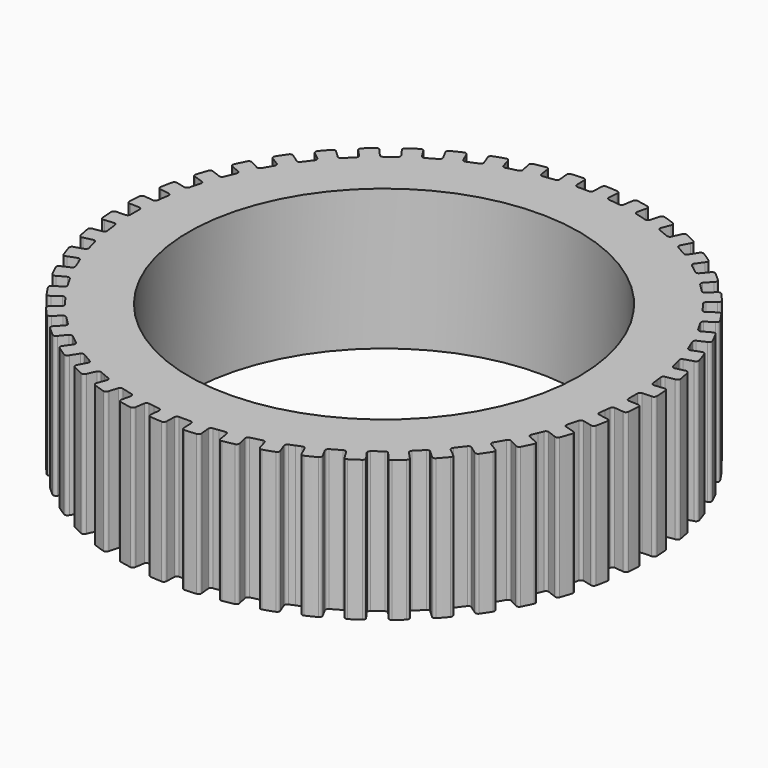
from build123d import *

# Parameters (mm, degrees)
F1_R     = 15
F1_R_2   = 11.1
F4_DEPTH = 8
F5_DEPTH = 8


# Not quite as in the source:
# - a feature names something its author has since deleted; it is built from what else it names


with BuildPart() as f4:
    # F1 (on Top) → F4 (new body)
    with BuildSketch(Plane.XY):
        Circle(F1_R)
        Circle(F1_R_2, mode=Mode.SUBTRACT)
    extrude(amount=F4_DEPTH)

    # F3 (on Top) + F2 (on Top) → F5 (cut)
    with BuildSketch(Plane.XY):
        with BuildLine():
            ThreePointArc((-14.6078107321, 2.4209827202), (-14.7318517717, 2.472566232), (-14.7728614863, 2.6004929356))
            Line((-14.7728614863, 2.6004929356), (-15.0180485763, 2.6327724283))
            Line((-15.0180485763, 2.6327724283), (-15.1877326262, 1.3438941086))
            Line((-15.1877326262, 1.3438941086), (-14.9425455361, 1.3116146158))
            ThreePointArc((-14.9425455361, 1.3116146158), (-14.8698233264, 1.4245682275), (-14.7366580875, 1.4422898902))
            Line((-14.7366580875, 1.4422898902), (-14.2148778682, 1.3912227941))
            ThreePointArc((-14.2148778682, 1.3912227941), (-14.1185132817, 1.4351704239), (-14.0707131699, 1.5296832643))
            Line((-14.0707131699, 1.5296832643), (-14.0289447884, 1.8469456199))
            Line((-14.0289447884, 1.8469456199), (-13.9871764069, 2.1642079756))
            ThreePointArc((-13.9871764069, 2.1642079756), (-14.0088860463, 2.2678719483), (-14.0905926055, 2.3352630891))
            Line((-14.0905926055, 2.3352630891), (-14.6078107321, 2.4209827202))
        make_face()
        with BuildLine():
            ThreePointArc((-13.4834652158, 6.1192693592), (-13.5899288642, 6.2011993888), (-13.5964313394, 6.3353811908))
            Line((-13.5964313394, 6.3353811908), (-13.8249093344, 6.4300198751))
            Line((-13.8249093344, 6.4300198751), (-14.3223977965, 5.2289764828))
            Line((-14.3223977965, 5.2289764828), (-14.0939198015, 5.1343377986))
            ThreePointArc((-14.0939198015, 5.1343377986), (-13.994440995, 5.2246207164), (-13.8612265478, 5.2072728282))
            Line((-13.8612265478, 5.2072728282), (-13.3704426953, 5.022899143))
            ThreePointArc((-13.3704426953, 5.022899143), (-13.265987169, 5.0404083034), (-13.1953540834, 5.1193291176))
            Line((-13.1953540834, 5.1193291176), (-13.072895385, 5.414970568))
            Line((-13.072895385, 5.414970568), (-12.9504366867, 5.7106120184))
            ThreePointArc((-12.9504366867, 5.7106120184), (-12.9445763776, 5.816362595), (-13.0060567426, 5.9026046521))
            Line((-13.0060567426, 5.9026046521), (-13.4834652158, 6.1192693592))
        make_face()
        with BuildLine():
            ThreePointArc((-14.4223273272, -3.3534707665), (-14.5566664602, -3.3532822666), (-14.6435099262, -3.2507871418))
            Line((-14.6435099262, -3.2507871418), (-14.8823860874, -3.3147938163))
            Line((-14.8823860874, -3.3147938163), (-14.5459213288, -4.5704973905))
            Line((-14.5459213288, -4.5704973905), (-14.3070451676, -4.506490716))
            ThreePointArc((-14.3070451676, -4.506490716), (-14.2830840823, -4.3743056012), (-14.1668372303, -4.306972789))
            Line((-14.1668372303, -4.306972789), (-13.6652326336, -4.1544759886))
            ThreePointArc((-13.6652326336, -4.1544759886), (-13.5930213943, -4.0769965423), (-13.5850283476, -3.9713857526))
            Line((-13.5850283476, -3.9713857526), (-13.667850442, -3.6622894882))
            Line((-13.667850442, -3.6622894882), (-13.7506725364, -3.3531932238))
            ThreePointArc((-13.7506725364, -3.3531932238), (-13.8104001128, -3.2657281204), (-13.9116766036, -3.2347345712))
            Line((-13.9116766036, -3.2347345712), (-14.4223273272, -3.3534707665))
        make_face()
        with BuildLine():
            ThreePointArc((-14.1668372303, 4.306972789), (-14.2830840823, 4.3743056012), (-14.3070451676, 4.506490716))
            Line((-14.3070451676, 4.506490716), (-14.5459213288, 4.5704973905))
            Line((-14.5459213288, 4.5704973905), (-14.8823860874, 3.3147938163))
            Line((-14.8823860874, 3.3147938163), (-14.6435099262, 3.2507871418))
            ThreePointArc((-14.6435099262, 3.2507871418), (-14.5566664602, 3.3532822666), (-14.4223273272, 3.3534707665))
            Line((-14.4223273272, 3.3534707665), (-13.9116766036, 3.2347345712))
            ThreePointArc((-13.9116766036, 3.2347345712), (-13.8104001128, 3.2657281204), (-13.7506725364, 3.3531932238))
            Line((-13.7506725364, 3.3531932238), (-13.667850442, 3.6622894882))
            Line((-13.667850442, 3.6622894882), (-13.5850283476, 3.9713857526))
            ThreePointArc((-13.5850283476, 3.9713857526), (-13.5930213943, 4.0769965423), (-13.6652326336, 4.1544759886))
            Line((-13.6652326336, 4.1544759886), (-14.1668372303, 4.306972789))
        make_face()
        with BuildLine():
            ThreePointArc((-14.7366580875, -1.4422898902), (-14.8698233264, -1.4245682275), (-14.9425455361, -1.3116146158))
            Line((-14.9425455361, -1.3116146158), (-15.1877326262, -1.3438941086))
            Line((-15.1877326262, -1.3438941086), (-15.0180485763, -2.6327724283))
            Line((-15.0180485763, -2.6327724283), (-14.7728614863, -2.6004929356))
            ThreePointArc((-14.7728614863, -2.6004929356), (-14.7318517717, -2.472566232), (-14.6078107321, -2.4209827202))
            Line((-14.6078107321, -2.4209827202), (-14.0905926055, -2.3352630891))
            ThreePointArc((-14.0905926055, -2.3352630891), (-14.0088860463, -2.2678719483), (-13.9871764069, -2.1642079756))
            Line((-13.9871764069, -2.1642079756), (-14.0289447884, -1.8469456199))
            Line((-14.0289447884, -1.8469456199), (-14.0707131699, -1.5296832643))
            ThreePointArc((-14.0707131699, -1.5296832643), (-14.1185132817, -1.4351704239), (-14.2148778682, -1.3912227941))
            Line((-14.2148778682, -1.3912227941), (-14.7366580875, -1.4422898902))
        make_face()
        with BuildLine():
            ThreePointArc((-14.7988405421, 0.4935689659), (-14.9285533928, 0.528520569), (-14.9859100491, 0.65))
            Line((-14.9859100491, 0.65), (-15.2332128489, 0.65))
            Line((-15.2332128489, 0.65), (-15.2332128489, -0.65))
            Line((-15.2332128489, -0.65), (-14.9859100491, -0.65))
            ThreePointArc((-14.9859100491, -0.65), (-14.9285533928, -0.528520569), (-14.7988405421, -0.4935689659))
            Line((-14.7988405421, -0.4935689659), (-14.2748586313, -0.4760931908))
            ThreePointArc((-14.2748586313, -0.4760931908), (-14.185054774, -0.4199434365), (-14.15, -0.32))
            Line((-14.15, -0.32), (-14.15, 0))
            Line((-14.15, 0), (-14.15, 0.32))
            ThreePointArc((-14.15, 0.32), (-14.185054774, 0.4199434365), (-14.2748586313, 0.4760931908))
            Line((-14.2748586313, 0.4760931908), (-14.7988405421, 0.4935689659))
        make_face()
        with BuildLine():
            ThreePointArc((-11.4402438275, 9.4005379039), (-11.5218747631, 9.5072310552), (-11.4934268659, 9.6385236877))
            Line((-11.4934268659, 9.6385236877), (-11.6896253682, 9.7890720935))
            Line((-11.6896253682, 9.7890720935), (-12.4810152259, 8.7577127511))
            Line((-12.4810152259, 8.7577127511), (-12.2848167236, 8.6071643453))
            ThreePointArc((-12.2848167236, 8.6071643453), (-12.1653606367, 8.6686239376), (-12.0411753256, 8.6173887283))
            Line((-12.0411753256, 8.6173887283), (-11.6148339485, 8.3122732161))
            ThreePointArc((-11.6148339485, 8.3122732161), (-11.5094059537, 8.3021506867), (-11.4207534224, 8.3601011516))
            Line((-11.4207534224, 8.3601011516), (-11.2259497651, 8.6139742205))
            Line((-11.2259497651, 8.6139742205), (-11.0311461078, 8.8678472894))
            ThreePointArc((-11.0311461078, 8.8678472894), (-10.9981152207, 8.9684777429), (-11.0351796062, 9.0676934625))
            Line((-11.0351796062, 9.0676934625), (-11.4402438275, 9.4005379039))
        make_face()
        with BuildLine():
            ThreePointArc((-10.1153545383, 10.8133664638), (-10.182360859, 10.9298018157), (-10.1370192102, 11.0562580257))
            Line((-10.1370192102, 11.0562580257), (-10.3118886969, 11.2311275125))
            Line((-10.3118886969, 11.2311275125), (-11.2311275125, 10.3118886969))
            Line((-11.2311275125, 10.3118886969), (-11.0562580257, 10.1370192102))
            ThreePointArc((-11.0562580257, 10.1370192102), (-10.9298018157, 10.182360859), (-10.8133664638, 10.1153545383))
            Line((-10.8133664638, 10.1153545383), (-10.4304980623, 9.757200615))
            ThreePointArc((-10.4304980623, 9.757200615), (-10.3272932739, 9.7334035705), (-10.2318351238, 9.7792867838))
            Line((-10.2318351238, 9.7792867838), (-10.0055609538, 10.0055609538))
            Line((-10.0055609538, 10.0055609538), (-9.7792867838, 10.2318351238))
            ThreePointArc((-9.7792867838, 10.2318351238), (-9.7334035705, 10.3272932739), (-9.757200615, 10.4304980623))
            Line((-9.757200615, 10.4304980623), (-10.1153545383, 10.8133664638))
        make_face()
        with BuildLine():
            ThreePointArc((-12.5693873731, 7.8268635341), (-12.6642461954, 7.9219889356), (-12.6531788014, 8.055871537))
            Line((-12.6531788014, 8.055871537), (-12.8673493084, 8.1795229369))
            Line((-12.8673493084, 8.1795229369), (-13.5173493084, 7.053689912))
            Line((-13.5173493084, 7.053689912), (-13.3031788014, 6.9300385121))
            ThreePointArc((-13.3031788014, 6.9300385121), (-13.1927667644, 7.0065644572), (-13.062956339, 6.9719770081))
            Line((-13.062956339, 6.9719770081), (-12.6004368055, 6.7251205179))
            ThreePointArc((-12.6004368055, 6.7251205179), (-12.4945895066, 6.7288457028), (-12.4142594635, 6.7978718708))
            Line((-12.4142594635, 6.7978718708), (-12.2542594635, 7.075))
            Line((-12.2542594635, 7.075), (-12.0942594635, 7.3521281292))
            ThreePointArc((-12.0942594635, 7.3521281292), (-12.0746460701, 7.4562090712), (-12.1243436147, 7.5497381134))
            Line((-12.1243436147, 7.5497381134), (-12.5693873731, 7.8268635341))
        make_face()
        with BuildLine():
            ThreePointArc((-8.6173887283, 12.0411753256), (-8.6686239376, 12.1653606367), (-8.6071643453, 12.2848167236))
            Line((-8.6071643453, 12.2848167236), (-8.7577127511, 12.4810152259))
            Line((-8.7577127511, 12.4810152259), (-9.7890720935, 11.6896253682))
            Line((-9.7890720935, 11.6896253682), (-9.6385236877, 11.4934268659))
            ThreePointArc((-9.6385236877, 11.4934268659), (-9.5072310552, 11.5218747631), (-9.4005379039, 11.4402438275))
            Line((-9.4005379039, 11.4402438275), (-9.0676934625, 11.0351796062))
            ThreePointArc((-9.0676934625, 11.0351796062), (-8.9684777429, 10.9981152207), (-8.8678472894, 11.0311461078))
            Line((-8.8678472894, 11.0311461078), (-8.6139742205, 11.2259497651))
            Line((-8.6139742205, 11.2259497651), (-8.3601011516, 11.4207534224))
            ThreePointArc((-8.3601011516, 11.4207534224), (-8.3021506867, 11.5094059537), (-8.3122732161, 11.6148339485))
            Line((-8.3122732161, 11.6148339485), (-8.6173887283, 12.0411753256))
        make_face()
        with BuildLine():
            ThreePointArc((-6.9719770081, 13.062956339), (-7.0065644572, 13.1927667644), (-6.9300385121, 13.3031788014))
            Line((-6.9300385121, 13.3031788014), (-7.053689912, 13.5173493084))
            Line((-7.053689912, 13.5173493084), (-8.1795229369, 12.8673493084))
            Line((-8.1795229369, 12.8673493084), (-8.055871537, 12.6531788014))
            ThreePointArc((-8.055871537, 12.6531788014), (-7.9219889356, 12.6642461954), (-7.8268635341, 12.5693873731))
            Line((-7.8268635341, 12.5693873731), (-7.5497381134, 12.1243436147))
            ThreePointArc((-7.5497381134, 12.1243436147), (-7.4562090712, 12.0746460701), (-7.3521281292, 12.0942594635))
            Line((-7.3521281292, 12.0942594635), (-7.075, 12.2542594635))
            Line((-7.075, 12.2542594635), (-6.7978718708, 12.4142594635))
            ThreePointArc((-6.7978718708, 12.4142594635), (-6.7288457028, 12.4945895066), (-6.7251205179, 12.6004368055))
            Line((-6.7251205179, 12.6004368055), (-6.9719770081, 13.062956339))
        make_face()
        with BuildLine():
            ThreePointArc((-5.2072728282, 13.8612265478), (-5.2246207164, 13.994440995), (-5.1343377986, 14.0939198015))
            Line((-5.1343377986, 14.0939198015), (-5.2289764828, 14.3223977965))
            Line((-5.2289764828, 14.3223977965), (-6.4300198751, 13.8249093344))
            Line((-6.4300198751, 13.8249093344), (-6.3353811908, 13.5964313394))
            ThreePointArc((-6.3353811908, 13.5964313394), (-6.2011993888, 13.5899288642), (-6.1192693592, 13.4834652158))
            Line((-6.1192693592, 13.4834652158), (-5.9026046521, 13.0060567426))
            ThreePointArc((-5.9026046521, 13.0060567426), (-5.816362595, 12.9445763776), (-5.7106120184, 12.9504366867))
            Line((-5.7106120184, 12.9504366867), (-5.414970568, 13.072895385))
            Line((-5.414970568, 13.072895385), (-5.1193291176, 13.1953540834))
            ThreePointArc((-5.1193291176, 13.1953540834), (-5.0404083034, 13.265987169), (-5.022899143, 13.3704426953))
            Line((-5.022899143, 13.3704426953), (-5.2072728282, 13.8612265478))
        make_face()
        with BuildLine():
            ThreePointArc((-1.4422898902, 14.7366580875), (-1.4245682275, 14.8698233264), (-1.3116146158, 14.9425455361))
            Line((-1.3116146158, 14.9425455361), (-1.3438941086, 15.1877326262))
            Line((-1.3438941086, 15.1877326262), (-2.6327724283, 15.0180485763))
            Line((-2.6327724283, 15.0180485763), (-2.6004929356, 14.7728614863))
            ThreePointArc((-2.6004929356, 14.7728614863), (-2.472566232, 14.7318517717), (-2.4209827202, 14.6078107321))
            Line((-2.4209827202, 14.6078107321), (-2.3352630891, 14.0905926055))
            ThreePointArc((-2.3352630891, 14.0905926055), (-2.2678719483, 14.0088860463), (-2.1642079756, 13.9871764069))
            Line((-2.1642079756, 13.9871764069), (-1.8469456199, 14.0289447884))
            Line((-1.8469456199, 14.0289447884), (-1.5296832643, 14.0707131699))
            ThreePointArc((-1.5296832643, 14.0707131699), (-1.4351704239, 14.1185132817), (-1.3912227941, 14.2148778682))
            Line((-1.3912227941, 14.2148778682), (-1.4422898902, 14.7366580875))
        make_face()
        with BuildLine():
            ThreePointArc((-3.3534707665, 14.4223273272), (-3.3532822666, 14.5566664602), (-3.2507871418, 14.6435099262))
            Line((-3.2507871418, 14.6435099262), (-3.3147938163, 14.8823860874))
            Line((-3.3147938163, 14.8823860874), (-4.5704973905, 14.5459213288))
            Line((-4.5704973905, 14.5459213288), (-4.506490716, 14.3070451676))
            ThreePointArc((-4.506490716, 14.3070451676), (-4.3743056012, 14.2830840823), (-4.306972789, 14.1668372303))
            Line((-4.306972789, 14.1668372303), (-4.1544759886, 13.6652326336))
            ThreePointArc((-4.1544759886, 13.6652326336), (-4.0769965423, 13.5930213943), (-3.9713857526, 13.5850283476))
            Line((-3.9713857526, 13.5850283476), (-3.6622894882, 13.667850442))
            Line((-3.6622894882, 13.667850442), (-3.3531932238, 13.7506725364))
            ThreePointArc((-3.3531932238, 13.7506725364), (-3.2657281204, 13.8104001128), (-3.2347345712, 13.9116766036))
            Line((-3.2347345712, 13.9116766036), (-3.3534707665, 14.4223273272))
        make_face()
        with BuildLine():
            Line((7.5497381134, 12.1243436147), (7.8268635341, 12.5693873731))
            ThreePointArc((7.8268635341, 12.5693873731), (7.9219889356, 12.6642461954), (8.055871537, 12.6531788014))
            Line((8.055871537, 12.6531788014), (8.1795229369, 12.8673493084))
            Line((8.1795229369, 12.8673493084), (7.053689912, 13.5173493084))
            Line((7.053689912, 13.5173493084), (6.9300385121, 13.3031788014))
            ThreePointArc((6.9300385121, 13.3031788014), (7.0065644572, 13.1927667644), (6.9719770081, 13.062956339))
            Line((6.9719770081, 13.062956339), (6.7251205179, 12.6004368055))
            ThreePointArc((6.7251205179, 12.6004368055), (6.7288457028, 12.4945895066), (6.7978718708, 12.4142594635))
            Line((6.7978718708, 12.4142594635), (7.075, 12.2542594635))
            Line((7.075, 12.2542594635), (7.3521281292, 12.0942594635))
            ThreePointArc((7.3521281292, 12.0942594635), (7.4562090712, 12.0746460701), (7.5497381134, 12.1243436147))
        make_face()
        with BuildLine():
            Line((10.4304980623, 9.757200615), (10.8133664638, 10.1153545383))
            ThreePointArc((10.8133664638, 10.1153545383), (10.9298018157, 10.182360859), (11.0562580257, 10.1370192102))
            Line((11.0562580257, 10.1370192102), (11.2311275125, 10.3118886969))
            Line((11.2311275125, 10.3118886969), (10.3118886969, 11.2311275125))
            Line((10.3118886969, 11.2311275125), (10.1370192102, 11.0562580257))
            ThreePointArc((10.1370192102, 11.0562580257), (10.182360859, 10.9298018157), (10.1153545383, 10.8133664638))
            Line((10.1153545383, 10.8133664638), (9.757200615, 10.4304980623))
            ThreePointArc((9.757200615, 10.4304980623), (9.7334035705, 10.3272932739), (9.7792867838, 10.2318351238))
            Line((9.7792867838, 10.2318351238), (10.0055609538, 10.0055609538))
            Line((10.0055609538, 10.0055609538), (10.2318351238, 9.7792867838))
            ThreePointArc((10.2318351238, 9.7792867838), (10.3272932739, 9.7334035705), (10.4304980623, 9.757200615))
        make_face()
        with BuildLine():
            Line((12.6004368055, 6.7251205179), (13.062956339, 6.9719770081))
            ThreePointArc((13.062956339, 6.9719770081), (13.1927667644, 7.0065644572), (13.3031788014, 6.9300385121))
            Line((13.3031788014, 6.9300385121), (13.5173493084, 7.053689912))
            Line((13.5173493084, 7.053689912), (12.8673493084, 8.1795229369))
            Line((12.8673493084, 8.1795229369), (12.6531788014, 8.055871537))
            ThreePointArc((12.6531788014, 8.055871537), (12.6642461954, 7.9219889356), (12.5693873731, 7.8268635341))
            Line((12.5693873731, 7.8268635341), (12.1243436147, 7.5497381134))
            ThreePointArc((12.1243436147, 7.5497381134), (12.0746460701, 7.4562090712), (12.0942594635, 7.3521281292))
            Line((12.0942594635, 7.3521281292), (12.2542594635, 7.075))
            Line((12.2542594635, 7.075), (12.4142594635, 6.7978718708))
            ThreePointArc((12.4142594635, 6.7978718708), (12.4945895066, 6.7288457028), (12.6004368055, 6.7251205179))
        make_face()
        with BuildLine():
            Line((9.0676934625, 11.0351796062), (9.4005379039, 11.4402438275))
            ThreePointArc((9.4005379039, 11.4402438275), (9.5072310552, 11.5218747631), (9.6385236877, 11.4934268659))
            Line((9.6385236877, 11.4934268659), (9.7890720935, 11.6896253682))
            Line((9.7890720935, 11.6896253682), (8.7577127511, 12.4810152259))
            Line((8.7577127511, 12.4810152259), (8.6071643453, 12.2848167236))
            ThreePointArc((8.6071643453, 12.2848167236), (8.6686239376, 12.1653606367), (8.6173887283, 12.0411753256))
            Line((8.6173887283, 12.0411753256), (8.3122732161, 11.6148339485))
            ThreePointArc((8.3122732161, 11.6148339485), (8.3021506867, 11.5094059537), (8.3601011516, 11.4207534224))
            Line((8.3601011516, 11.4207534224), (8.6139742205, 11.2259497651))
            Line((8.6139742205, 11.2259497651), (8.8678472894, 11.0311461078))
            ThreePointArc((8.8678472894, 11.0311461078), (8.9684777429, 10.9981152207), (9.0676934625, 11.0351796062))
        make_face()
        with BuildLine():
            Line((13.3704426953, 5.022899143), (13.8612265478, 5.2072728282))
            ThreePointArc((13.8612265478, 5.2072728282), (13.994440995, 5.2246207164), (14.0939198015, 5.1343377986))
            Line((14.0939198015, 5.1343377986), (14.3223977965, 5.2289764828))
            Line((14.3223977965, 5.2289764828), (13.8249093344, 6.4300198751))
            Line((13.8249093344, 6.4300198751), (13.5964313394, 6.3353811908))
            ThreePointArc((13.5964313394, 6.3353811908), (13.5899288642, 6.2011993888), (13.4834652158, 6.1192693592))
            Line((13.4834652158, 6.1192693592), (13.0060567426, 5.9026046521))
            ThreePointArc((13.0060567426, 5.9026046521), (12.9445763776, 5.816362595), (12.9504366867, 5.7106120184))
            Line((12.9504366867, 5.7106120184), (13.072895385, 5.414970568))
            Line((13.072895385, 5.414970568), (13.1953540834, 5.1193291176))
            ThreePointArc((13.1953540834, 5.1193291176), (13.265987169, 5.0404083034), (13.3704426953, 5.022899143))
        make_face()
        with BuildLine():
            Line((11.6148339485, 8.3122732161), (12.0411753256, 8.6173887283))
            ThreePointArc((12.0411753256, 8.6173887283), (12.1653606367, 8.6686239376), (12.2848167236, 8.6071643453))
            Line((12.2848167236, 8.6071643453), (12.4810152259, 8.7577127511))
            Line((12.4810152259, 8.7577127511), (11.6896253682, 9.7890720935))
            Line((11.6896253682, 9.7890720935), (11.4934268659, 9.6385236877))
            ThreePointArc((11.4934268659, 9.6385236877), (11.5218747631, 9.5072310552), (11.4402438275, 9.4005379039))
            Line((11.4402438275, 9.4005379039), (11.0351796062, 9.0676934625))
            ThreePointArc((11.0351796062, 9.0676934625), (10.9981152207, 8.9684777429), (11.0311461078, 8.8678472894))
            Line((11.0311461078, 8.8678472894), (11.2259497651, 8.6139742205))
            Line((11.2259497651, 8.6139742205), (11.4207534224, 8.3601011516))
            ThreePointArc((11.4207534224, 8.3601011516), (11.5094059537, 8.3021506867), (11.6148339485, 8.3122732161))
        make_face()
        with BuildLine():
            Line((13.9116766036, 3.2347345712), (14.4223273272, 3.3534707665))
            ThreePointArc((14.4223273272, 3.3534707665), (14.5566664602, 3.3532822666), (14.6435099262, 3.2507871418))
            Line((14.6435099262, 3.2507871418), (14.8823860874, 3.3147938163))
            Line((14.8823860874, 3.3147938163), (14.5459213288, 4.5704973905))
            Line((14.5459213288, 4.5704973905), (14.3070451676, 4.506490716))
            ThreePointArc((14.3070451676, 4.506490716), (14.2830840823, 4.3743056012), (14.1668372303, 4.306972789))
            Line((14.1668372303, 4.306972789), (13.6652326336, 4.1544759886))
            ThreePointArc((13.6652326336, 4.1544759886), (13.5930213943, 4.0769965423), (13.5850283476, 3.9713857526))
            Line((13.5850283476, 3.9713857526), (13.667850442, 3.6622894882))
            Line((13.667850442, 3.6622894882), (13.7506725364, 3.3531932238))
            ThreePointArc((13.7506725364, 3.3531932238), (13.8104001128, 3.2657281204), (13.9116766036, 3.2347345712))
        make_face()
        with BuildLine():
            ThreePointArc((14.6078107321, -2.4209827202), (14.7318517717, -2.472566232), (14.7728614863, -2.6004929356))
            Line((14.7728614863, -2.6004929356), (15.0180485763, -2.6327724283))
            Line((15.0180485763, -2.6327724283), (15.1877326262, -1.3438941086))
            Line((15.1877326262, -1.3438941086), (14.9425455361, -1.3116146158))
            ThreePointArc((14.9425455361, -1.3116146158), (14.8698233264, -1.4245682275), (14.7366580875, -1.4422898902))
            Line((14.7366580875, -1.4422898902), (14.2148778682, -1.3912227941))
            ThreePointArc((14.2148778682, -1.3912227941), (14.1185132817, -1.4351704239), (14.0707131699, -1.5296832643))
            Line((14.0707131699, -1.5296832643), (14.0289447884, -1.8469456199))
            Line((14.0289447884, -1.8469456199), (13.9871764069, -2.1642079756))
            ThreePointArc((13.9871764069, -2.1642079756), (14.0088860463, -2.2678719483), (14.0905926055, -2.3352630891))
            Line((14.0905926055, -2.3352630891), (14.6078107321, -2.4209827202))
        make_face()
        with BuildLine():
            Line((14.2748586313, -0.4760931908), (14.7988405421, -0.4935689659))
            ThreePointArc((14.7988405421, -0.4935689659), (14.9285533928, -0.528520569), (14.9859100491, -0.65))
            Line((14.9859100491, -0.65), (15.2332128489, -0.65))
            Line((15.2332128489, -0.65), (15.2332128489, 0.65))
            Line((15.2332128489, 0.65), (14.9859100491, 0.65))
            ThreePointArc((14.9859100491, 0.65), (14.9285533928, 0.528520569), (14.7988405421, 0.4935689659))
            Line((14.7988405421, 0.4935689659), (14.2748586313, 0.4760931908))
            ThreePointArc((14.2748586313, 0.4760931908), (14.185054774, 0.4199434365), (14.15, 0.32))
            Line((14.15, 0.32), (14.15, 0))
            Line((14.15, 0), (14.15, -0.32))
            ThreePointArc((14.15, -0.32), (14.185054774, -0.4199434365), (14.2748586313, -0.4760931908))
        make_face()
        with BuildLine():
            Line((14.2148778682, 1.3912227941), (14.7366580875, 1.4422898902))
            ThreePointArc((14.7366580875, 1.4422898902), (14.8698233264, 1.4245682275), (14.9425455361, 1.3116146158))
            Line((14.9425455361, 1.3116146158), (15.1877326262, 1.3438941086))
            Line((15.1877326262, 1.3438941086), (15.0180485763, 2.6327724283))
            Line((15.0180485763, 2.6327724283), (14.7728614863, 2.6004929356))
            ThreePointArc((14.7728614863, 2.6004929356), (14.7318517717, 2.472566232), (14.6078107321, 2.4209827202))
            Line((14.6078107321, 2.4209827202), (14.0905926055, 2.3352630891))
            ThreePointArc((14.0905926055, 2.3352630891), (14.0088860463, 2.2678719483), (13.9871764069, 2.1642079756))
            Line((13.9871764069, 2.1642079756), (14.0289447884, 1.8469456199))
            Line((14.0289447884, 1.8469456199), (14.0707131699, 1.5296832643))
            ThreePointArc((14.0707131699, 1.5296832643), (14.1185132817, 1.4351704239), (14.2148778682, 1.3912227941))
        make_face()
        with BuildLine():
            ThreePointArc((-13.8612265478, -5.2072728282), (-13.994440995, -5.2246207164), (-14.0939198015, -5.1343377986))
            Line((-14.0939198015, -5.1343377986), (-14.3223977965, -5.2289764828))
            Line((-14.3223977965, -5.2289764828), (-13.8249093344, -6.4300198751))
            Line((-13.8249093344, -6.4300198751), (-13.5964313394, -6.3353811908))
            ThreePointArc((-13.5964313394, -6.3353811908), (-13.5899288642, -6.2011993888), (-13.4834652158, -6.1192693592))
            Line((-13.4834652158, -6.1192693592), (-13.0060567426, -5.9026046521))
            ThreePointArc((-13.0060567426, -5.9026046521), (-12.9445763776, -5.816362595), (-12.9504366867, -5.7106120184))
            Line((-12.9504366867, -5.7106120184), (-13.072895385, -5.414970568))
            Line((-13.072895385, -5.414970568), (-13.1953540834, -5.1193291176))
            ThreePointArc((-13.1953540834, -5.1193291176), (-13.265987169, -5.0404083034), (-13.3704426953, -5.022899143))
            Line((-13.3704426953, -5.022899143), (-13.8612265478, -5.2072728282))
        make_face()
        with BuildLine():
            ThreePointArc((-13.062956339, -6.9719770081), (-13.1927667644, -7.0065644572), (-13.3031788014, -6.9300385121))
            Line((-13.3031788014, -6.9300385121), (-13.5173493084, -7.053689912))
            Line((-13.5173493084, -7.053689912), (-12.8673493084, -8.1795229369))
            Line((-12.8673493084, -8.1795229369), (-12.6531788014, -8.055871537))
            ThreePointArc((-12.6531788014, -8.055871537), (-12.6642461954, -7.9219889356), (-12.5693873731, -7.8268635341))
            Line((-12.5693873731, -7.8268635341), (-12.1243436147, -7.5497381134))
            ThreePointArc((-12.1243436147, -7.5497381134), (-12.0746460701, -7.4562090712), (-12.0942594635, -7.3521281292))
            Line((-12.0942594635, -7.3521281292), (-12.2542594635, -7.075))
            Line((-12.2542594635, -7.075), (-12.4142594635, -6.7978718708))
            ThreePointArc((-12.4142594635, -6.7978718708), (-12.4945895066, -6.7288457028), (-12.6004368055, -6.7251205179))
            Line((-12.6004368055, -6.7251205179), (-13.062956339, -6.9719770081))
        make_face()
        with BuildLine():
            ThreePointArc((-12.0411753256, -8.6173887283), (-12.1653606367, -8.6686239376), (-12.2848167236, -8.6071643453))
            Line((-12.2848167236, -8.6071643453), (-12.4810152259, -8.7577127511))
            Line((-12.4810152259, -8.7577127511), (-11.6896253682, -9.7890720935))
            Line((-11.6896253682, -9.7890720935), (-11.4934268659, -9.6385236877))
            ThreePointArc((-11.4934268659, -9.6385236877), (-11.5218747631, -9.5072310552), (-11.4402438275, -9.4005379039))
            Line((-11.4402438275, -9.4005379039), (-11.0351796062, -9.0676934625))
            ThreePointArc((-11.0351796062, -9.0676934625), (-10.9981152207, -8.9684777429), (-11.0311461078, -8.8678472894))
            Line((-11.0311461078, -8.8678472894), (-11.2259497651, -8.6139742205))
            Line((-11.2259497651, -8.6139742205), (-11.4207534224, -8.3601011516))
            ThreePointArc((-11.4207534224, -8.3601011516), (-11.5094059537, -8.3021506867), (-11.6148339485, -8.3122732161))
            Line((-11.6148339485, -8.3122732161), (-12.0411753256, -8.6173887283))
        make_face()
        with BuildLine():
            ThreePointArc((-9.4005379039, -11.4402438275), (-9.5072310552, -11.5218747631), (-9.6385236877, -11.4934268659))
            Line((-9.6385236877, -11.4934268659), (-9.7890720935, -11.6896253682))
            Line((-9.7890720935, -11.6896253682), (-8.7577127511, -12.4810152259))
            Line((-8.7577127511, -12.4810152259), (-8.6071643453, -12.2848167236))
            ThreePointArc((-8.6071643453, -12.2848167236), (-8.6686239376, -12.1653606367), (-8.6173887283, -12.0411753256))
            Line((-8.6173887283, -12.0411753256), (-8.3122732161, -11.6148339485))
            ThreePointArc((-8.3122732161, -11.6148339485), (-8.3021506867, -11.5094059537), (-8.3601011516, -11.4207534224))
            Line((-8.3601011516, -11.4207534224), (-8.6139742205, -11.2259497651))
            Line((-8.6139742205, -11.2259497651), (-8.8678472894, -11.0311461078))
            ThreePointArc((-8.8678472894, -11.0311461078), (-8.9684777429, -10.9981152207), (-9.0676934625, -11.0351796062))
            Line((-9.0676934625, -11.0351796062), (-9.4005379039, -11.4402438275))
        make_face()
        with BuildLine():
            ThreePointArc((-7.8268635341, -12.5693873731), (-7.9219889356, -12.6642461954), (-8.055871537, -12.6531788014))
            Line((-8.055871537, -12.6531788014), (-8.1795229369, -12.8673493084))
            Line((-8.1795229369, -12.8673493084), (-7.053689912, -13.5173493084))
            Line((-7.053689912, -13.5173493084), (-6.9300385121, -13.3031788014))
            ThreePointArc((-6.9300385121, -13.3031788014), (-7.0065644572, -13.1927667644), (-6.9719770081, -13.062956339))
            Line((-6.9719770081, -13.062956339), (-6.7251205179, -12.6004368055))
            ThreePointArc((-6.7251205179, -12.6004368055), (-6.7288457028, -12.4945895066), (-6.7978718708, -12.4142594635))
            Line((-6.7978718708, -12.4142594635), (-7.075, -12.2542594635))
            Line((-7.075, -12.2542594635), (-7.3521281292, -12.0942594635))
            ThreePointArc((-7.3521281292, -12.0942594635), (-7.4562090712, -12.0746460701), (-7.5497381134, -12.1243436147))
            Line((-7.5497381134, -12.1243436147), (-7.8268635341, -12.5693873731))
        make_face()
        with BuildLine():
            ThreePointArc((-10.8133664638, -10.1153545383), (-10.9298018157, -10.182360859), (-11.0562580257, -10.1370192102))
            Line((-11.0562580257, -10.1370192102), (-11.2311275125, -10.3118886969))
            Line((-11.2311275125, -10.3118886969), (-10.3118886969, -11.2311275125))
            Line((-10.3118886969, -11.2311275125), (-10.1370192102, -11.0562580257))
            ThreePointArc((-10.1370192102, -11.0562580257), (-10.182360859, -10.9298018157), (-10.1153545383, -10.8133664638))
            Line((-10.1153545383, -10.8133664638), (-9.757200615, -10.4304980623))
            ThreePointArc((-9.757200615, -10.4304980623), (-9.7334035705, -10.3272932739), (-9.7792867838, -10.2318351238))
            Line((-9.7792867838, -10.2318351238), (-10.0055609538, -10.0055609538))
            Line((-10.0055609538, -10.0055609538), (-10.2318351238, -9.7792867838))
            ThreePointArc((-10.2318351238, -9.7792867838), (-10.3272932739, -9.7334035705), (-10.4304980623, -9.757200615))
            Line((-10.4304980623, -9.757200615), (-10.8133664638, -10.1153545383))
        make_face()
        with BuildLine():
            ThreePointArc((-6.1192693592, -13.4834652158), (-6.2011993888, -13.5899288642), (-6.3353811908, -13.5964313394))
            Line((-6.3353811908, -13.5964313394), (-6.4300198751, -13.8249093344))
            Line((-6.4300198751, -13.8249093344), (-5.2289764828, -14.3223977965))
            Line((-5.2289764828, -14.3223977965), (-5.1343377986, -14.0939198015))
            ThreePointArc((-5.1343377986, -14.0939198015), (-5.2246207164, -13.994440995), (-5.2072728282, -13.8612265478))
            Line((-5.2072728282, -13.8612265478), (-5.022899143, -13.3704426953))
            ThreePointArc((-5.022899143, -13.3704426953), (-5.0404083034, -13.265987169), (-5.1193291176, -13.1953540834))
            Line((-5.1193291176, -13.1953540834), (-5.414970568, -13.072895385))
            Line((-5.414970568, -13.072895385), (-5.7106120184, -12.9504366867))
            ThreePointArc((-5.7106120184, -12.9504366867), (-5.816362595, -12.9445763776), (-5.9026046521, -13.0060567426))
            Line((-5.9026046521, -13.0060567426), (-6.1192693592, -13.4834652158))
        make_face()
        with BuildLine():
            ThreePointArc((-4.306972789, -14.1668372303), (-4.3743056012, -14.2830840823), (-4.506490716, -14.3070451676))
            Line((-4.506490716, -14.3070451676), (-4.5704973905, -14.5459213288))
            Line((-4.5704973905, -14.5459213288), (-3.3147938163, -14.8823860874))
            Line((-3.3147938163, -14.8823860874), (-3.2507871418, -14.6435099262))
            ThreePointArc((-3.2507871418, -14.6435099262), (-3.3532822666, -14.5566664602), (-3.3534707665, -14.4223273272))
            Line((-3.3534707665, -14.4223273272), (-3.2347345712, -13.9116766036))
            ThreePointArc((-3.2347345712, -13.9116766036), (-3.2657281204, -13.8104001128), (-3.3531932238, -13.7506725364))
            Line((-3.3531932238, -13.7506725364), (-3.6622894882, -13.667850442))
            Line((-3.6622894882, -13.667850442), (-3.9713857526, -13.5850283476))
            ThreePointArc((-3.9713857526, -13.5850283476), (-4.0769965423, -13.5930213943), (-4.1544759886, -13.6652326336))
            Line((-4.1544759886, -13.6652326336), (-4.306972789, -14.1668372303))
        make_face()
        with BuildLine():
            ThreePointArc((-2.4209827202, -14.6078107321), (-2.472566232, -14.7318517717), (-2.6004929356, -14.7728614863))
            Line((-2.6004929356, -14.7728614863), (-2.6327724283, -15.0180485763))
            Line((-2.6327724283, -15.0180485763), (-1.3438941086, -15.1877326262))
            Line((-1.3438941086, -15.1877326262), (-1.3116146158, -14.9425455361))
            ThreePointArc((-1.3116146158, -14.9425455361), (-1.4245682275, -14.8698233264), (-1.4422898902, -14.7366580875))
            Line((-1.4422898902, -14.7366580875), (-1.3912227941, -14.2148778682))
            ThreePointArc((-1.3912227941, -14.2148778682), (-1.4351704239, -14.1185132817), (-1.5296832643, -14.0707131699))
            Line((-1.5296832643, -14.0707131699), (-1.8469456199, -14.0289447884))
            Line((-1.8469456199, -14.0289447884), (-2.1642079756, -13.9871764069))
            ThreePointArc((-2.1642079756, -13.9871764069), (-2.2678719483, -14.0088860463), (-2.3352630891, -14.0905926055))
            Line((-2.3352630891, -14.0905926055), (-2.4209827202, -14.6078107321))
        make_face()
        with BuildLine():
            ThreePointArc((-0.4935689659, -14.7988405421), (-0.528520569, -14.9285533928), (-0.65, -14.9859100491))
            Line((-0.65, -14.9859100491), (-0.65, -15.2332128489))
            Line((-0.65, -15.2332128489), (0.65, -15.2332128489))
            Line((0.65, -15.2332128489), (0.65, -14.9859100491))
            ThreePointArc((0.65, -14.9859100491), (0.528520569, -14.9285533928), (0.4935689659, -14.7988405421))
            Line((0.4935689659, -14.7988405421), (0.4760931908, -14.2748586313))
            ThreePointArc((0.4760931908, -14.2748586313), (0.4199434365, -14.185054774), (0.32, -14.15))
            Line((0.32, -14.15), (0, -14.15))
            Line((0, -14.15), (-0.32, -14.15))
            ThreePointArc((-0.32, -14.15), (-0.4199434365, -14.185054774), (-0.4760931908, -14.2748586313))
            Line((-0.4760931908, -14.2748586313), (-0.4935689659, -14.7988405421))
        make_face()
        with BuildLine():
            ThreePointArc((1.4422898902, -14.7366580875), (1.4245682275, -14.8698233264), (1.3116146158, -14.9425455361))
            Line((1.3116146158, -14.9425455361), (1.3438941086, -15.1877326262))
            Line((1.3438941086, -15.1877326262), (2.6327724283, -15.0180485763))
            Line((2.6327724283, -15.0180485763), (2.6004929356, -14.7728614863))
            ThreePointArc((2.6004929356, -14.7728614863), (2.472566232, -14.7318517717), (2.4209827202, -14.6078107321))
            Line((2.4209827202, -14.6078107321), (2.3352630891, -14.0905926055))
            ThreePointArc((2.3352630891, -14.0905926055), (2.2678719483, -14.0088860463), (2.1642079756, -13.9871764069))
            Line((2.1642079756, -13.9871764069), (1.8469456199, -14.0289447884))
            Line((1.8469456199, -14.0289447884), (1.5296832643, -14.0707131699))
            ThreePointArc((1.5296832643, -14.0707131699), (1.4351704239, -14.1185132817), (1.3912227941, -14.2148778682))
            Line((1.3912227941, -14.2148778682), (1.4422898902, -14.7366580875))
        make_face()
        with BuildLine():
            ThreePointArc((3.3534707665, -14.4223273272), (3.3532822666, -14.5566664602), (3.2507871418, -14.6435099262))
            Line((3.2507871418, -14.6435099262), (3.3147938163, -14.8823860874))
            Line((3.3147938163, -14.8823860874), (4.5704973905, -14.5459213288))
            Line((4.5704973905, -14.5459213288), (4.506490716, -14.3070451676))
            ThreePointArc((4.506490716, -14.3070451676), (4.3743056012, -14.2830840823), (4.306972789, -14.1668372303))
            Line((4.306972789, -14.1668372303), (4.1544759886, -13.6652326336))
            ThreePointArc((4.1544759886, -13.6652326336), (4.0769965423, -13.5930213943), (3.9713857526, -13.5850283476))
            Line((3.9713857526, -13.5850283476), (3.6622894882, -13.667850442))
            Line((3.6622894882, -13.667850442), (3.3531932238, -13.7506725364))
            ThreePointArc((3.3531932238, -13.7506725364), (3.2657281204, -13.8104001128), (3.2347345712, -13.9116766036))
            Line((3.2347345712, -13.9116766036), (3.3534707665, -14.4223273272))
        make_face()
        with BuildLine():
            ThreePointArc((5.2072728282, -13.8612265478), (5.2246207164, -13.994440995), (5.1343377986, -14.0939198015))
            Line((5.1343377986, -14.0939198015), (5.2289764828, -14.3223977965))
            Line((5.2289764828, -14.3223977965), (6.4300198751, -13.8249093344))
            Line((6.4300198751, -13.8249093344), (6.3353811908, -13.5964313394))
            ThreePointArc((6.3353811908, -13.5964313394), (6.2011993888, -13.5899288642), (6.1192693592, -13.4834652158))
            Line((6.1192693592, -13.4834652158), (5.9026046521, -13.0060567426))
            ThreePointArc((5.9026046521, -13.0060567426), (5.816362595, -12.9445763776), (5.7106120184, -12.9504366867))
            Line((5.7106120184, -12.9504366867), (5.414970568, -13.072895385))
            Line((5.414970568, -13.072895385), (5.1193291176, -13.1953540834))
            ThreePointArc((5.1193291176, -13.1953540834), (5.0404083034, -13.265987169), (5.022899143, -13.3704426953))
            Line((5.022899143, -13.3704426953), (5.2072728282, -13.8612265478))
        make_face()
        with BuildLine():
            ThreePointArc((6.9719770081, -13.062956339), (7.0065644572, -13.1927667644), (6.9300385121, -13.3031788014))
            Line((6.9300385121, -13.3031788014), (7.053689912, -13.5173493084))
            Line((7.053689912, -13.5173493084), (8.1795229369, -12.8673493084))
            Line((8.1795229369, -12.8673493084), (8.055871537, -12.6531788014))
            ThreePointArc((8.055871537, -12.6531788014), (7.9219889356, -12.6642461954), (7.8268635341, -12.5693873731))
            Line((7.8268635341, -12.5693873731), (7.5497381134, -12.1243436147))
            ThreePointArc((7.5497381134, -12.1243436147), (7.4562090712, -12.0746460701), (7.3521281292, -12.0942594635))
            Line((7.3521281292, -12.0942594635), (7.075, -12.2542594635))
            Line((7.075, -12.2542594635), (6.7978718708, -12.4142594635))
            ThreePointArc((6.7978718708, -12.4142594635), (6.7288457028, -12.4945895066), (6.7251205179, -12.6004368055))
            Line((6.7251205179, -12.6004368055), (6.9719770081, -13.062956339))
        make_face()
        with BuildLine():
            ThreePointArc((8.6173887283, -12.0411753256), (8.6686239376, -12.1653606367), (8.6071643453, -12.2848167236))
            Line((8.6071643453, -12.2848167236), (8.7577127511, -12.4810152259))
            Line((8.7577127511, -12.4810152259), (9.7890720935, -11.6896253682))
            Line((9.7890720935, -11.6896253682), (9.6385236877, -11.4934268659))
            ThreePointArc((9.6385236877, -11.4934268659), (9.5072310552, -11.5218747631), (9.4005379039, -11.4402438275))
            Line((9.4005379039, -11.4402438275), (9.0676934625, -11.0351796062))
            ThreePointArc((9.0676934625, -11.0351796062), (8.9684777429, -10.9981152207), (8.8678472894, -11.0311461078))
            Line((8.8678472894, -11.0311461078), (8.6139742205, -11.2259497651))
            Line((8.6139742205, -11.2259497651), (8.3601011516, -11.4207534224))
            ThreePointArc((8.3601011516, -11.4207534224), (8.3021506867, -11.5094059537), (8.3122732161, -11.6148339485))
            Line((8.3122732161, -11.6148339485), (8.6173887283, -12.0411753256))
        make_face()
        with BuildLine():
            ThreePointArc((10.1153545383, -10.8133664638), (10.182360859, -10.9298018157), (10.1370192102, -11.0562580257))
            Line((10.1370192102, -11.0562580257), (10.3118886969, -11.2311275125))
            Line((10.3118886969, -11.2311275125), (11.2311275125, -10.3118886969))
            Line((11.2311275125, -10.3118886969), (11.0562580257, -10.1370192102))
            ThreePointArc((11.0562580257, -10.1370192102), (10.9298018157, -10.182360859), (10.8133664638, -10.1153545383))
            Line((10.8133664638, -10.1153545383), (10.4304980623, -9.757200615))
            ThreePointArc((10.4304980623, -9.757200615), (10.3272932739, -9.7334035705), (10.2318351238, -9.7792867838))
            Line((10.2318351238, -9.7792867838), (10.0055609538, -10.0055609538))
            Line((10.0055609538, -10.0055609538), (9.7792867838, -10.2318351238))
            ThreePointArc((9.7792867838, -10.2318351238), (9.7334035705, -10.3272932739), (9.757200615, -10.4304980623))
            Line((9.757200615, -10.4304980623), (10.1153545383, -10.8133664638))
        make_face()
        with BuildLine():
            ThreePointArc((11.4402438275, -9.4005379039), (11.5218747631, -9.5072310552), (11.4934268659, -9.6385236877))
            Line((11.4934268659, -9.6385236877), (11.6896253682, -9.7890720935))
            Line((11.6896253682, -9.7890720935), (12.4810152259, -8.7577127511))
            Line((12.4810152259, -8.7577127511), (12.2848167236, -8.6071643453))
            ThreePointArc((12.2848167236, -8.6071643453), (12.1653606367, -8.6686239376), (12.0411753256, -8.6173887283))
            Line((12.0411753256, -8.6173887283), (11.6148339485, -8.3122732161))
            ThreePointArc((11.6148339485, -8.3122732161), (11.5094059537, -8.3021506867), (11.4207534224, -8.3601011516))
            Line((11.4207534224, -8.3601011516), (11.2259497651, -8.6139742205))
            Line((11.2259497651, -8.6139742205), (11.0311461078, -8.8678472894))
            ThreePointArc((11.0311461078, -8.8678472894), (10.9981152207, -8.9684777429), (11.0351796062, -9.0676934625))
            Line((11.0351796062, -9.0676934625), (11.4402438275, -9.4005379039))
        make_face()
        with BuildLine():
            ThreePointArc((12.5693873731, -7.8268635341), (12.6642461954, -7.9219889356), (12.6531788014, -8.055871537))
            Line((12.6531788014, -8.055871537), (12.8673493084, -8.1795229369))
            Line((12.8673493084, -8.1795229369), (13.5173493084, -7.053689912))
            Line((13.5173493084, -7.053689912), (13.3031788014, -6.9300385121))
            ThreePointArc((13.3031788014, -6.9300385121), (13.1927667644, -7.0065644572), (13.062956339, -6.9719770081))
            Line((13.062956339, -6.9719770081), (12.6004368055, -6.7251205179))
            ThreePointArc((12.6004368055, -6.7251205179), (12.4945895066, -6.7288457028), (12.4142594635, -6.7978718708))
            Line((12.4142594635, -6.7978718708), (12.2542594635, -7.075))
            Line((12.2542594635, -7.075), (12.0942594635, -7.3521281292))
            ThreePointArc((12.0942594635, -7.3521281292), (12.0746460701, -7.4562090712), (12.1243436147, -7.5497381134))
            Line((12.1243436147, -7.5497381134), (12.5693873731, -7.8268635341))
        make_face()
        with BuildLine():
            ThreePointArc((13.4834652158, -6.1192693592), (13.5899288642, -6.2011993888), (13.5964313394, -6.3353811908))
            Line((13.5964313394, -6.3353811908), (13.8249093344, -6.4300198751))
            Line((13.8249093344, -6.4300198751), (14.3223977965, -5.2289764828))
            Line((14.3223977965, -5.2289764828), (14.0939198015, -5.1343377986))
            ThreePointArc((14.0939198015, -5.1343377986), (13.994440995, -5.2246207164), (13.8612265478, -5.2072728282))
            Line((13.8612265478, -5.2072728282), (13.3704426953, -5.022899143))
            ThreePointArc((13.3704426953, -5.022899143), (13.265987169, -5.0404083034), (13.1953540834, -5.1193291176))
            Line((13.1953540834, -5.1193291176), (13.072895385, -5.414970568))
            Line((13.072895385, -5.414970568), (12.9504366867, -5.7106120184))
            ThreePointArc((12.9504366867, -5.7106120184), (12.9445763776, -5.816362595), (13.0060567426, -5.9026046521))
            Line((13.0060567426, -5.9026046521), (13.4834652158, -6.1192693592))
        make_face()
        with BuildLine():
            ThreePointArc((14.1668372303, -4.306972789), (14.2830840823, -4.3743056012), (14.3070451676, -4.506490716))
            Line((14.3070451676, -4.506490716), (14.5459213288, -4.5704973905))
            Line((14.5459213288, -4.5704973905), (14.8823860874, -3.3147938163))
            Line((14.8823860874, -3.3147938163), (14.6435099262, -3.2507871418))
            ThreePointArc((14.6435099262, -3.2507871418), (14.5566664602, -3.3532822666), (14.4223273272, -3.3534707665))
            Line((14.4223273272, -3.3534707665), (13.9116766036, -3.2347345712))
            ThreePointArc((13.9116766036, -3.2347345712), (13.8104001128, -3.2657281204), (13.7506725364, -3.3531932238))
            Line((13.7506725364, -3.3531932238), (13.667850442, -3.6622894882))
            Line((13.667850442, -3.6622894882), (13.5850283476, -3.9713857526))
            ThreePointArc((13.5850283476, -3.9713857526), (13.5930213943, -4.0769965423), (13.6652326336, -4.1544759886))
            Line((13.6652326336, -4.1544759886), (14.1668372303, -4.306972789))
        make_face()
        with BuildLine():
            Line((2.3352630891, 14.0905926055), (2.4209827202, 14.6078107321))
            ThreePointArc((2.4209827202, 14.6078107321), (2.472566232, 14.7318517717), (2.6004929356, 14.7728614863))
            Line((2.6004929356, 14.7728614863), (2.6327724283, 15.0180485763))
            Line((2.6327724283, 15.0180485763), (1.3438941086, 15.1877326262))
            Line((1.3438941086, 15.1877326262), (1.3116146158, 14.9425455361))
            ThreePointArc((1.3116146158, 14.9425455361), (1.4245682275, 14.8698233264), (1.4422898902, 14.7366580875))
            Line((1.4422898902, 14.7366580875), (1.3912227941, 14.2148778682))
            ThreePointArc((1.3912227941, 14.2148778682), (1.4351704239, 14.1185132817), (1.5296832643, 14.0707131699))
            Line((1.5296832643, 14.0707131699), (1.8469456199, 14.0289447884))
            Line((1.8469456199, 14.0289447884), (2.1642079756, 13.9871764069))
            ThreePointArc((2.1642079756, 13.9871764069), (2.2678719483, 14.0088860463), (2.3352630891, 14.0905926055))
        make_face()
        with BuildLine():
            Line((4.1544759886, 13.6652326336), (4.306972789, 14.1668372303))
            ThreePointArc((4.306972789, 14.1668372303), (4.3743056012, 14.2830840823), (4.506490716, 14.3070451676))
            Line((4.506490716, 14.3070451676), (4.5704973905, 14.5459213288))
            Line((4.5704973905, 14.5459213288), (3.3147938163, 14.8823860874))
            Line((3.3147938163, 14.8823860874), (3.2507871418, 14.6435099262))
            ThreePointArc((3.2507871418, 14.6435099262), (3.3532822666, 14.5566664602), (3.3534707665, 14.4223273272))
            Line((3.3534707665, 14.4223273272), (3.2347345712, 13.9116766036))
            ThreePointArc((3.2347345712, 13.9116766036), (3.2657281204, 13.8104001128), (3.3531932238, 13.7506725364))
            Line((3.3531932238, 13.7506725364), (3.6622894882, 13.667850442))
            Line((3.6622894882, 13.667850442), (3.9713857526, 13.5850283476))
            ThreePointArc((3.9713857526, 13.5850283476), (4.0769965423, 13.5930213943), (4.1544759886, 13.6652326336))
        make_face()
        with BuildLine():
            Line((5.9026046521, 13.0060567426), (6.1192693592, 13.4834652158))
            ThreePointArc((6.1192693592, 13.4834652158), (6.2011993888, 13.5899288642), (6.3353811908, 13.5964313394))
            Line((6.3353811908, 13.5964313394), (6.4300198751, 13.8249093344))
            Line((6.4300198751, 13.8249093344), (5.2289764828, 14.3223977965))
            Line((5.2289764828, 14.3223977965), (5.1343377986, 14.0939198015))
            ThreePointArc((5.1343377986, 14.0939198015), (5.2246207164, 13.994440995), (5.2072728282, 13.8612265478))
            Line((5.2072728282, 13.8612265478), (5.022899143, 13.3704426953))
            ThreePointArc((5.022899143, 13.3704426953), (5.0404083034, 13.265987169), (5.1193291176, 13.1953540834))
            Line((5.1193291176, 13.1953540834), (5.414970568, 13.072895385))
            Line((5.414970568, 13.072895385), (5.7106120184, 12.9504366867))
            ThreePointArc((5.7106120184, 12.9504366867), (5.816362595, 12.9445763776), (5.9026046521, 13.0060567426))
        make_face()
    with BuildSketch(Plane.XY):
        with BuildLine():
            ThreePointArc((-0.65, 14.9859100491), (0, 15), (0.65, 14.9859100491))
            Line((0.65, 14.9859100491), (0.65, 15.2332128489))
            Line((0.65, 15.2332128489), (-0.65, 15.2332128489))
            Line((-0.65, 15.2332128489), (-0.65, 14.9859100491))
        make_face()
        with BuildLine():
            ThreePointArc((0.4935689659, 14.7988405421), (0.528520569, 14.9285533928), (0.65, 14.9859100491))
            ThreePointArc((0.65, 14.9859100491), (0, 15), (-0.65, 14.9859100491))
            ThreePointArc((-0.65, 14.9859100491), (-0.528520569, 14.9285533928), (-0.4935689659, 14.7988405421))
            Line((-0.4935689659, 14.7988405421), (-0.4760931908, 14.2748586313))
            ThreePointArc((-0.4760931908, 14.2748586313), (-0.4199434365, 14.185054774), (-0.32, 14.15))
            Line((-0.32, 14.15), (0, 14.15))
            Line((0, 14.15), (0.32, 14.15))
            ThreePointArc((0.32, 14.15), (0.4199434365, 14.185054774), (0.4760931908, 14.2748586313))
            Line((0.4760931908, 14.2748586313), (0.4935689659, 14.7988405421))
        make_face()
    extrude(amount=F5_DEPTH, mode=Mode.SUBTRACT)


solid = f4.part
